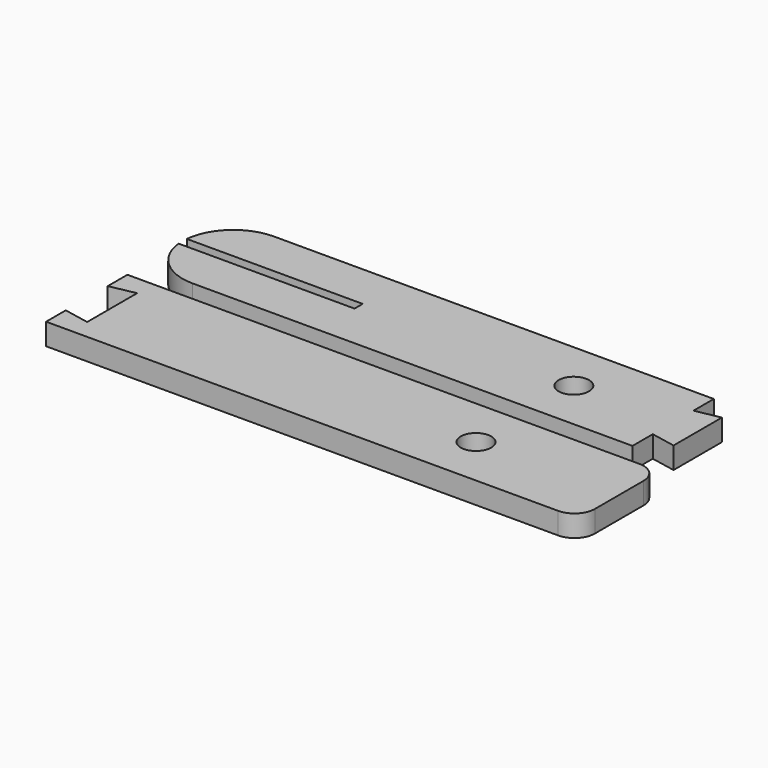
from build123d import *

# Parameters (mm, degrees)
F1_DEPTH     = 6.35
F2_DEPTH     = 6.35
F6_TEXT_SIZE = 18.584743763
F7_DEPTH     = 1.25
F8_DEPTH     = 0.4
F10_DEPTH    = 6.75


# Not quite as in the source:
# - Text() gives the source's letters only with a copy of the font that has no kerning and outlines rounded to 1/6400 em; it was checked with that copy


with BuildPart() as f1:
    # F0 (on Top) → F1 (new body)
    with BuildSketch(Plane.XY):
        with BuildLine():
            ThreePointArc((-31.5299411752, 0), (-26.7799411752, 4.75), (-22.0299411752, 0))
            Line((-22.0299411752, 0), (11.8639487773, 0))
            Line((11.8639487773, 0), (11.8639487773, 9.430273436))
            Line((11.8639487773, 9.430273436), (4.1950992309, 7.9248))
            Line((4.1950992309, 7.9248), (4.1950992309, 15.8496))
            Line((4.1950992309, 15.8496), (-132.9519411752, 15.8496))
            ThreePointArc((-132.9519411752, 15.8496), (-143.5832294358, 11.7552341567), (-148.7218385722, 1.5875))
            Line((-148.7218385722, 1.5875), (-93.8740411752, 1.5875))
            Line((-93.8740411752, 1.5875), (-93.8740411752, 0))
            Line((-93.8740411752, 0), (-31.5299411752, 0))
        make_face()
        with BuildLine():
            Line((11.8639487773, 0), (-22.0299411752, 0))
            ThreePointArc((-22.0299411752, 0), (-26.7799411752, -4.75), (-31.5299411752, 0))
            Line((-31.5299411752, 0), (-93.8740411752, 0))
            Line((-93.8740411752, 0), (-93.8740411752, -1.5875))
            Line((-93.8740411752, -1.5875), (-148.7218385722, -1.5875))
            ThreePointArc((-148.7218385722, -1.5875), (-143.5832294358, -11.7552341567), (-132.9519411752, -15.8496))
            Line((-132.9519411752, -15.8496), (4.1950992309, -15.8496))
            Line((4.1950992309, -15.8496), (4.1950992309, -7.9248))
            Line((4.1950992309, -7.9248), (11.8639487773, -9.430273436))
            Line((11.8639487773, -9.430273436), (11.8639487773, 0))
        make_face()
    extrude(amount=F1_DEPTH)

    # F8 (add): a face of the model
    f8_faces = [f1.faces().sort_by_distance(p)[0] for p in [
        (-67.1431224107, 0, 6.35),
    ]]
    extrude(f8_faces, amount=F8_DEPTH)


with BuildPart() as f2:
    # F0 (on Top) → F2 (new body)
    with BuildSketch(Plane.XY):
        with BuildLine():
            Line((120.8192588248, 0), (28.9726480842, 0))
            Line((28.9726480842, 0), (28.9726480842, -15.8496))
            Line((28.9726480842, -15.8496), (163.8724588248, -15.8496))
            ThreePointArc((163.8724588248, -15.8496), (168.3625868853, -13.9897280605), (170.2224588248, -9.4996))
            Line((170.2224588248, -9.4996), (170.2224588248, 0))
            Line((170.2224588248, 0), (130.3192588248, 0))
            ThreePointArc((130.3192588248, 0), (125.5692588248, -4.75), (120.8192588248, 0))
        make_face()
        with BuildLine():
            Line((28.9726480842, 15.8496), (28.9726480842, 0))
            Line((28.9726480842, 0), (120.8192588248, 0))
            ThreePointArc((120.8192588248, 0), (125.5692588248, 4.75), (130.3192588248, 0))
            Line((130.3192588248, 0), (170.2224588248, 0))
            Line((170.2224588248, 0), (170.2224588248, 9.4996))
            ThreePointArc((170.2224588248, 9.4996), (168.3625868853, 13.9897280605), (163.8724588248, 15.8496))
            Line((163.8724588248, 15.8496), (28.9726480842, 15.8496))
        make_face()
        Polygon((28.9726480842, 0), (11.8639487773, 0), (11.8639487773, -9.430273436), (4.1950992309, -7.9248), (4.1950992309, -15.8496), (28.9726480842, -15.8496), align=None)
        Polygon((11.8639487773, 9.430273436), (11.8639487773, 0), (28.9726480842, 0), (28.9726480842, 15.8496), (4.1950992309, 15.8496), (4.1950992309, 7.9248), align=None)
    extrude(amount=F2_DEPTH)


with BuildPart() as f2_1:
    # F3: moved
    add(f2.part.moved(Location((0, -15.8496, 0))))


with BuildPart() as f2_2:
    # F4: moved
    add(f2_1.part.moved(Location((0, -15.8496, 0))))


with BuildPart() as f2_3:
    # F5: moved
    add(f2_2.part.moved(Location((-152.4, -6.35, 0))))

    # F6 (on face) → F7 (cut)
    with BuildSketch(Plane(origin=(0, 0, 0), x_dir=(1, 0, 0), z_dir=(0, 0, -1))):
        with Locations((-131.5355971456, 31.5817482769)):
            Text('MB  DN  CS', F6_TEXT_SIZE, font='Open Sans', text_align=(TextAlign.LEFT, TextAlign.BOTTOM))
    extrude(amount=-F7_DEPTH, mode=Mode.SUBTRACT)

    # F8#2 (add): a face of the model
    f8_2_faces = [f2_3.faces().sort_by_distance(p)[0] for p in [
        (-63.9233281641, -38.0492, 6.35),
    ]]
    extrude(f8_2_faces, amount=F8_DEPTH)

    # F9 (on face) → F10 (cut, through all)
    with BuildSketch(Plane.XY.offset(6.75)):
        Polygon((-148.2049007691, -29.8696283256), (-148.2049007691, -30.1244), (-140.5360512227, -28.618926564), (-140.5360512227, -47.479473436), (-148.2049007691, -45.974), (-148.2049007691, -46.2287716744), (-140.2860512227, -47.7833226619), (-140.2860512227, -28.3150773381), align=None)
    extrude(amount=-F10_DEPTH, mode=Mode.SUBTRACT)


solid = Compound([f1.part, f2_3.part])
